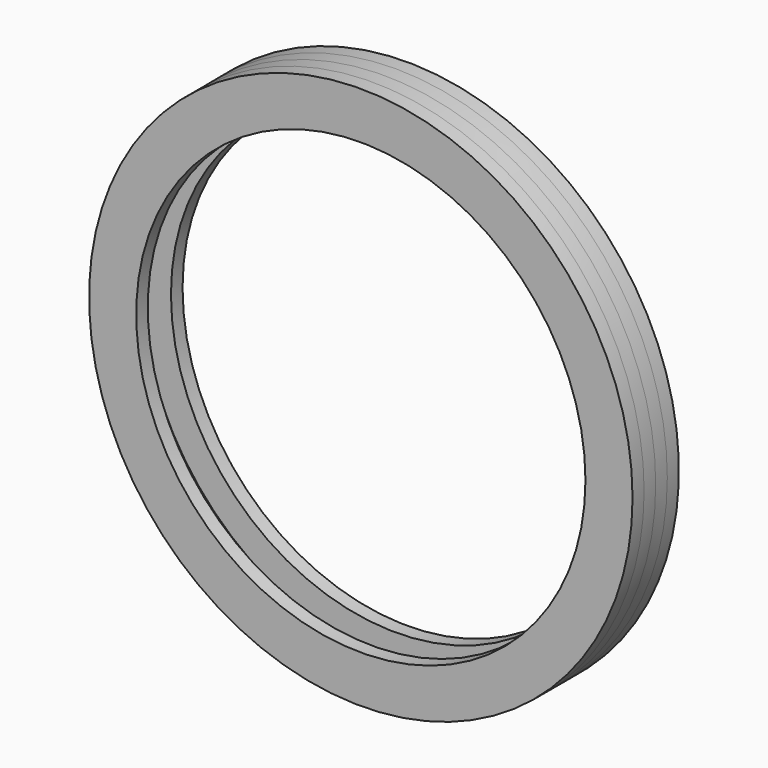
from build123d import *

# Parameters (mm, degrees)
F0_R          = 37.5
F0_R_2        = 35
F1_DEPTH      = 2
F1_DEPTH_BACK = 2
F2_R          = 37.5
F2_R_2        = 31
F3_DEPTH      = 2
F4_R          = 37.5
F4_R_2        = 31
F5_DEPTH      = 2


# Not quite as in the source:
# - a feature names something its author has since deleted; it is built from what else it names


with BuildPart() as f1:
    # F0 (on Front) → F1 (new body, two sides)
    with BuildSketch(Plane.XZ) as f1_sk:
        Circle(F0_R)
        Circle(F0_R_2, mode=Mode.SUBTRACT)
    extrude(amount=-F1_DEPTH)
    extrude(f1_sk.sketch, amount=F1_DEPTH_BACK)

    # F2 (on face) → F3 (join)
    with BuildSketch(Plane.XZ.offset(2)):
        Circle(F2_R)
        Circle(F2_R_2, mode=Mode.SUBTRACT)
    extrude(amount=F3_DEPTH)

    # F4 (on face) → F5 (join)
    with BuildSketch(Plane(origin=(0, 2, 0), x_dir=(-1, 0, 0), z_dir=(0, 1, 0))):
        Circle(F4_R)
        Circle(F4_R_2, mode=Mode.SUBTRACT)
    extrude(amount=F5_DEPTH)


solid = f1.part
